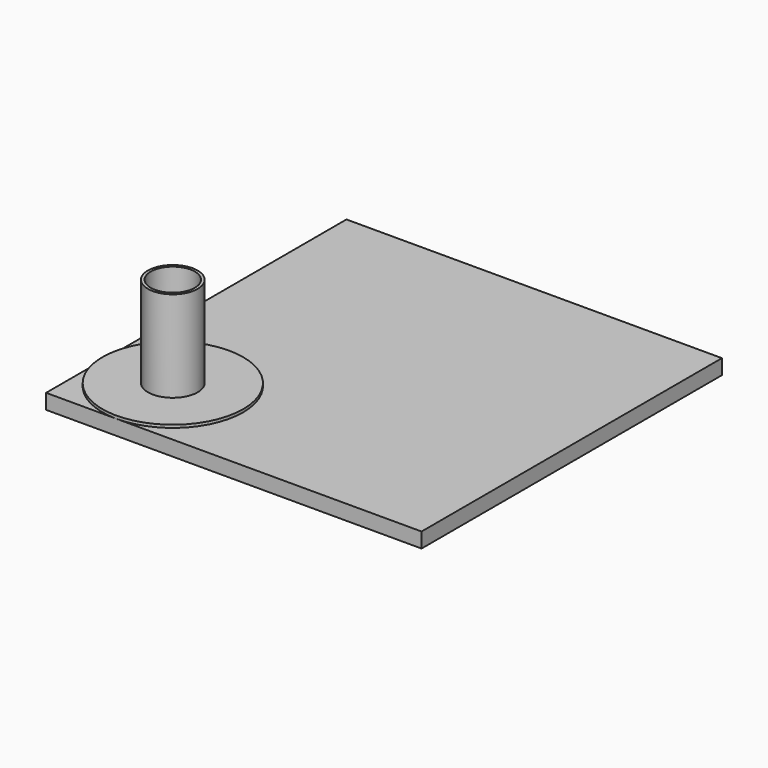
from build123d import *

# Parameters (mm, degrees)
F0_R     = 26.5
F1_DEPTH = 100
F2_T     = -3
F3_R     = 75
F4_DEPTH = 3
F5_W     = 400
F5_H     = 400
F6_DEPTH = 16


# Not quite as in the source:
# - a feature names something its author has since deleted; it is built from what else it names


with BuildPart() as f1:
    # F0 (on Top) → F1 (new body)
    with BuildSketch(Plane.XY):
        Circle(F0_R)
    extrude(amount=F1_DEPTH)

    # F2
    f2_openings = [f1.faces().sort_by_distance(p)[0] for p in [
        (0, 0, 100),
        (0, 0, 0),
    ]]
    offset(amount=F2_T, openings=f2_openings)

    # F3 (on Top) → F4 (join)
    with BuildSketch(Plane.XY):
        Circle(F3_R)
    extrude(amount=F4_DEPTH)

    # F5 (on Top) → F6 (join)
    with BuildSketch(Plane.XY):
        with Locations((125, 125)):
            Rectangle(F5_W, F5_H)
    extrude(amount=-F6_DEPTH)


solid = f1.part
